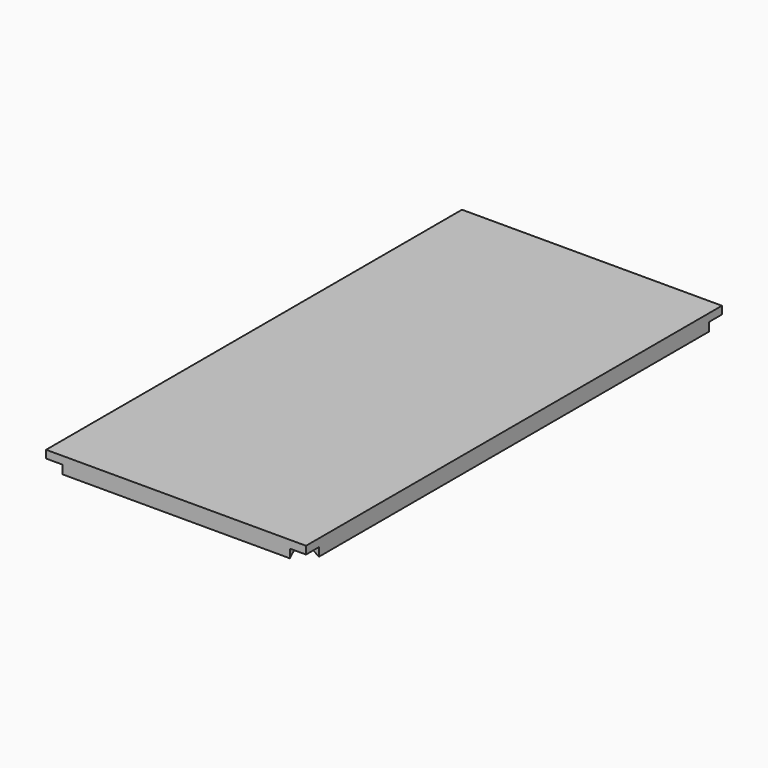
from build123d import *

# Parameters (mm, degrees)
F1_DEPTH = 203.2
F3_DEPTH = 44.45
F5_DEPTH = 6.35
F7_DEPTH = 6.35


# Not quite as in the source:
# - a pattern or mirror of a feature is missing from the dataset's text; its kind, count and spacing are read off the source's solid


with BuildPart() as f1:
    # F0 (on Front) → F1 (new body)
    with BuildSketch(Plane.XZ):
        Polygon((50.8, 0), (0, 0), (-50.8, 0), (-50.8, -6.35), (-45.386130618, -3.0314885393), (45.382719487, -3.0314885393), (50.8, -6.35), align=None)
    extrude(amount=F1_DEPTH)

    # F2 (on Right) → F3 (join, symmetric)
    with BuildSketch(Plane.YZ):
        Polygon((0, -6.3831382431), (0, 0), (-3.5511243623, 0), (-3.5511243623, -3.1539145857), align=None)
    f3 = extrude(amount=F3_DEPTH, both=True)

    # F3_copies: F3 across plane
    add(f3.mirror(Plane(origin=(0, -101.6, 0), x_dir=(0, 0, -1), z_dir=(0, -1, 0))))

    # F4 (on Front) → F5 (cut)
    with BuildSketch(Plane.XZ):
        Polygon((50.8, -3.0314885393), (45.382719487, -3.0314885393), (50.8, -6.35), align=None)
        Polygon((-50.8, -3.0314885393), (-50.8, -6.35), (-45.382719487, -3.0314885393), align=None)
    extrude(amount=F5_DEPTH, mode=Mode.SUBTRACT)

    # F6 (on face) → F7 (cut)
    with BuildSketch(Plane.XZ.offset(203.2)):
        Polygon((-50.8, -6.35), (-45.386130618, -3.0314885393), (-50.8, -3.0314885393), align=None)
        Polygon((50.8, -6.35), (50.8, -3.0314885393), (45.382719487, -3.0314885393), align=None)
    extrude(amount=-F7_DEPTH, mode=Mode.SUBTRACT)


solid = f1.part
